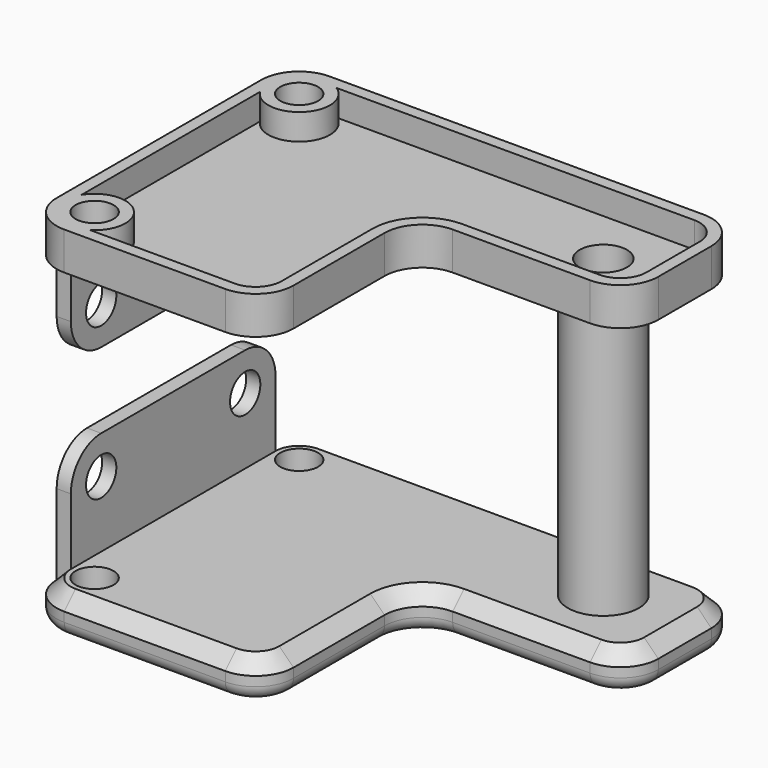
from build123d import *

# Parameters (mm, degrees)
F0_R         = 4
F1_DEPTH     = 8
F2_R         = 4
F3_DEPTH     = 3
F5_R         = 7.5
F6_DEPTH     = 60
F9_R         = 3
F10_SIZE     = 2.99999
F11_T        = 2.5
F11_T3_DEPTH = 5.00001
F11_T5_DEPTH = 59
F11_T7_DEPTH = 9.242626545
F11_T9_DEPTH = 8


# Not quite as in the source:
# - a fillet or chamfer is up to 0.001 mm smaller than in the source, because OpenCascade refuses the exact size
# - a shell that OpenCascade refuses in one call is made with other operations: the cavity is built on its own and cut out


with BuildPart() as f1:
    # F0 (on Top) → F1 (new body)
    with BuildSketch(Plane.XY):
        with BuildLine():
            Line((0, -32), (0, -8))
            ThreePointArc((0, -8), (2.3431457505, -2.3431457505), (8, 0))
            Line((8, 0), (37, 0))
            ThreePointArc((37, 0), (42.6568542495, 2.3431457505), (45, 8))
            Line((45, 8), (45, 22))
            ThreePointArc((45, 22), (42.6568542495, 27.6568542495), (37, 30))
            Line((37, 30), (-42, 30))
            ThreePointArc((-42, 30), (-47.6568542495, 27.6568542495), (-50, 22))
            Line((-50, 22), (-50, -32))
            ThreePointArc((-50, -32), (-47.6568542495, -37.6568542495), (-42, -40))
            Line((-42, -40), (-8, -40))
            ThreePointArc((-8, -40), (-2.3431457505, -37.6568542495), (0, -32))
        make_face()
        with Locations((-42, -32)):
            Circle(F0_R, mode=Mode.SUBTRACT)
        with Locations((-42, 22)):
            Circle(F0_R, mode=Mode.SUBTRACT)
    extrude(amount=F1_DEPTH)

    # F2 (on face) → F3 (join)
    with BuildSketch(Plane(origin=(-50, 0, 0), x_dir=(0, -1, 0), z_dir=(-1, 0, 0))):
        with BuildLine():
            Line((-22, 22), (-22, 8))
            Line((-22, 8), (32, 8))
            Line((32, 8), (32, 22))
            ThreePointArc((32, 22), (29.6568542495, 27.6568542495), (24, 30))
            Line((24, 30), (-14, 30))
            ThreePointArc((-14, 30), (-19.6568542495, 27.6568542495), (-22, 22))
        make_face()
        with Locations((-14, 22)):
            Circle(F2_R, mode=Mode.SUBTRACT)
        with Locations((24, 22)):
            Circle(F2_R, mode=Mode.SUBTRACT)
    extrude(amount=-F3_DEPTH)

    # F5 (on offset) → F6 (join, through all)
    with BuildSketch(Plane.XY.offset(68)):
        with Locations((27.2762235254, 15.6497936696)):
            Circle(F5_R)
    extrude(amount=-F6_DEPTH)

    # F8: F1 across plane


with BuildPart() as f1_1:
    add(f1.part)
    add(f1.part.mirror(Plane(origin=(-11.4052960318, 0.3495814809, 38), x_dir=(1, 0, 0), z_dir=(0, 0, 1))))

    # F9
    f9_edges = [f1_1.edges().sort_by_distance(p)[0] for p in [
        (-25, -40, 0),
        (0, -20, 0),
        (-2.343146, -37.656854, 0),
        (2.343146, -2.343146, 0),
        (22.5, 0, 0),
        (42.656854, 2.343146, 0),
        (45, 15, 0),
        (42.656854, 27.656854, 0),
        (-2.5, 30, 0),
        (-47.656854, 27.656854, 0),
        (-50, -5, 0),
        (-47.656854, -37.656854, 0),
    ]]
    fillet(f9_edges, radius=F9_R)

    # F10 (size 3 in the source; OpenCascade refuses exactly that, so slightly less here)
    f10_edges = [f1_1.edges().sort_by_distance(p)[0] for p in [
        (-25, -40, 8),
        (-2.343146, -37.656854, 8),
        (0, -20, 8),
        (-47.656854, -37.656854, 8),
        (2.343146, -2.343146, 8),
        (22.5, 0, 8),
        (42.656854, 2.343146, 8),
        (45, 15, 8),
        (-47.656854, 27.656854, 8),
        (42.656854, 27.656854, 8),
        (-2.5, 30, 8),
    ]]
    chamfer(f10_edges, length=F10_SIZE)

    # F11: shell of thickness 2.5, made by hand


with BuildPart() as f11_core1:
    # F11_t2: copy of F1
    add(f1_1.part)

    # the walls: a layer under each face that stays
    f11_faces = [f11_core1.faces().sort_by_distance(p)[0] for p in [
        (0, -20, 4.000005),
        (-2.3431457505, -37.6568542495, 4.000005),
        (-1.499995, -20, 6.500005),
        (-0.8786796564, -20, 0.8786796564),
        (2.3431457505, -2.3431457505, 4.000005),
        (-25, -40, 4.000005),
        (-3.4038023868, -36.5961976132, 6.500005),
        (-2.9644660941, -37.0355339059, 0.8786796564),
        (-32.1666733333, -26.33334, 8),
        (1.2824891143, -1.2824891143, 6.500005),
        (-32.1666666667, -26.3333333333, 0),
        (1.7218254069, -1.7218254069, 0.8786796564),
        (22.5, 0, 4.000005),
        (-47.6568542495, -37.6568542495, 4.000005),
        (-25, -38.500005, 6.500005),
        (-25, -39.1213203436, 0.8786796564),
        (-48.5, -32, 13.500005),
        (-46.5961976132, -36.5961976132, 6.500005),
        (-47, -5, 19),
        (-48.5, 22, 13.500005),
        (-46.5961976132, 26.5961976132, 6.500005),
        (-2.5, 28.500005, 6.500005),
        (41.5961976132, 26.5961976132, 6.500005),
        (22.5, 1.499995, 6.500005),
        (43.500005, 15, 6.500005),
        (41.5961976132, 3.4038023868, 6.500005),
        (-46, -32, 4),
        (-46, 22, 4),
        (19.7762235254, 15.6497936696, 38),
        (-47.0355339059, -37.0355339059, 0.8786796564),
        (-49.1213203436, -5, 0.8786796564),
        (-47.0355339059, 27.0355339059, 0.8786796564),
        (-2.5, 29.1213203436, 0.8786796564),
        (22.5, 0.8786796564, 0.8786796564),
        (42.0355339059, 27.0355339059, 0.8786796564),
        (42.0355339059, 2.9644660941, 0.8786796564),
        (44.1213203436, 15, 0.8786796564),
        (42.6568542495, 2.3431457505, 4.000005),
        (-50, -5, 16.5),
        (-48.5, -29.6568542495, 27.6568542495),
        (-48.5, -5, 30),
        (-48.5, 19.6568542495, 27.6568542495),
        (-48.5, 18, 22),
        (-48.5, -20, 22),
        (-47.6568542495, 27.6568542495, 4.000005),
        (-2.5, 30, 4.000005),
        (42.6568542495, 27.6568542495, 4.000005),
        (45, 15, 4.000005),
        (-2.5, -5, 68),
        (-2.3431457505, -37.6568542495, 72),
        (-25, -40, 72),
        (0, -20, 72),
        (-47.6568542495, -37.6568542495, 72),
        (2.3431457505, -2.3431457505, 72),
        (-48.5, -32, 61),
        (22.5, 0, 72),
        (-47, -5, 57),
        (42.6568542495, 2.3431457505, 72),
        (-48.5, 22, 61),
        (45, 15, 72),
        (-47.6568542495, 27.6568542495, 72),
        (42.6568542495, 27.6568542495, 72),
        (-2.5, 30, 72),
        (-46, -32, 72),
        (-46, 22, 72),
        (-50, -5, 61),
        (-48.5, -29.6568542495, 48.3431457505),
        (-48.5, -5, 46),
        (-48.5, 19.6568542495, 48.3431457505),
        (-48.5, 18, 54),
        (-48.5, -20, 54),
    ]]
    thicken(f11_faces, amount=-F11_T, mode=Mode.SUBTRACT)

    # F11_s4 → F11_t3 (cut)
    with BuildSketch(Plane.YZ.offset(-49.50001)):
        Polygon((-32.025, 8.025), (-32, 5.5), (-29.5, 5.5), (-29.5, 8), align=None)
        Polygon((22.025, 8.025), (22, 5.5), (19.5, 5.5), (19.5, 8), align=None)
    extrude(amount=F11_T3_DEPTH, mode=Mode.SUBTRACT)

    # F11_s6 → F11_t5 (cut)
    with BuildSketch(Plane.XZ.offset(-24.5)):
        Polygon((-46.975, 8.025), (-47, 5.5), (-49.5, 5.5), (-49.5, 8), align=None)
        Polygon((-46.975, 67.975), (-47, 70.5), (-49.5, 70.5), (-49.5, 68), align=None)
    extrude(amount=F11_T5_DEPTH, mode=Mode.SUBTRACT)

    # F11_s8 → F11_t7 (cut)
    with BuildSketch(Plane(origin=(-17.732238047, 0, -17.732238047), x_dir=(0, 1, 0), z_dir=(-0.7071067812, 0, -0.7071067812))):
        Polygon((-32.025, -38.9158800363), (-29.5, -38.8908800363), (-29.5, -36.3908800363), (-32, -36.3908800363), align=None)
        Polygon((22.025, -38.9158800363), (19.5, -38.8908800363), (19.5, -36.3908800363), (22, -36.3908800363), align=None)
    extrude(amount=F11_T7_DEPTH, mode=Mode.SUBTRACT)

    # F11_s10 → F11_t9 (cut)
    with BuildSketch(Plane.YZ.offset(-52.5)):
        Polygon((-32.025, 67.975), (-32, 70.5), (-29.5, 70.5), (-29.5, 68), align=None)
        Polygon((22.025, 67.975), (22, 70.5), (19.5, 70.5), (19.5, 68), align=None)
    extrude(amount=F11_T9_DEPTH, mode=Mode.SUBTRACT)

    # F11_s11 → F11_t12 (revolve, cut)
    with BuildSketch(Plane.XZ.offset(-15.6497936696)):
        Polygon((34.8012235254, 8.025), (34.7762235254, 5.5), (32.2762235254, 5.5), (32.2762235254, 8), align=None)
    revolve(axis=Axis((27.2762235254, 15.6497936696, 8), (0, 0, 1)), mode=Mode.SUBTRACT)

    # F11_s13 → F11_t14 (revolve, cut)
    with BuildSketch(Plane.XZ.offset(-15.6497936696)):
        Polygon((34.8012235254, 67.975), (32.2762235254, 68), (32.2762235254, 70.5), (34.7762235254, 70.5), align=None)
    revolve(axis=Axis((27.2762235254, 15.6497936696, 68), (0, 0, 1)), mode=Mode.SUBTRACT)


with BuildPart() as f1_2:
    add(f1_1.part)

    # what is left inside the walls is the cavity
    f11_cavity = [f11_core1.part.solids().sort_by_distance(p)[0] for p in [
        (-25, 5.833333, 75.975),
    ]]
    add(f11_cavity, mode=Mode.SUBTRACT)


solid = f1_2.part
